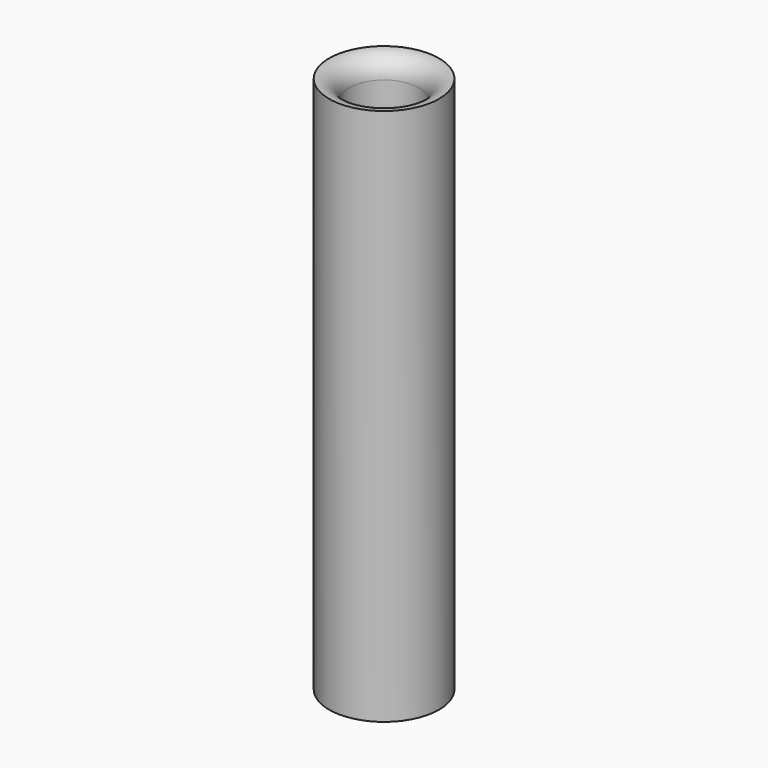
from build123d import *

# Parameters (mm, degrees)
F0_R     = 14
F0_R_2   = 9
F1_DEPTH = 137
F2_R     = 4.99999


# Not quite as in the source:
# - a fillet or chamfer is up to 0.001 mm smaller than in the source, because OpenCascade refuses the exact size


with BuildPart() as f1:
    # F0 (on Top) → F1 (new body)
    with BuildSketch(Plane.XY):
        Circle(F0_R)
        Circle(F0_R_2, mode=Mode.SUBTRACT)
    extrude(amount=F1_DEPTH)

    # F2 (radius 5 in the source; OpenCascade refuses exactly that, so slightly less here)
    f2_edges = [f1.edges().sort_by_distance(p)[0] for p in [
        (-9, 0, 137),
        (-9, 0, 0),
    ]]
    fillet(f2_edges, radius=F2_R)


solid = f1.part
